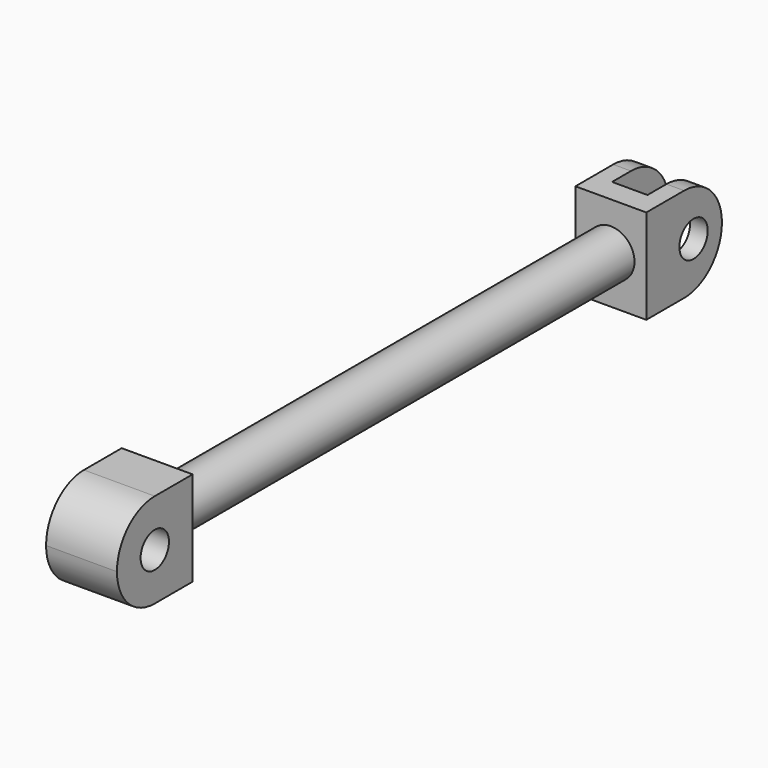
from build123d import *

# Parameters (mm, degrees)
F0_R      = 12.7
F1_DEPTH  = 304.8
F2_W      = 38.1
F2_H      = 50.8
F3_DEPTH  = 50.8
F4_R      = 9.525
F5_DEPTH  = 38.101
F6_W      = 38.1
F6_H      = 50.8
F7_DEPTH  = 50.8
F8_W      = 19.05
F8_H      = 50.8
F9_DEPTH  = 38.1
F10_R     = 9.525
F11_DEPTH = 38.101
F12_R     = 25.39999


# Not quite as in the source:
# - a fillet or chamfer is up to 0.001 mm smaller than in the source, because OpenCascade refuses the exact size


with BuildPart() as f1:
    # F0 (on Front) → F1 (new body)
    with BuildSketch(Plane.XZ):
        Circle(F0_R)
    extrude(amount=F1_DEPTH)

    # F2 (on face) → F3 (join)
    with BuildSketch(Plane.XZ.offset(304.8)):
        Rectangle(F2_W, F2_H)
    extrude(amount=F3_DEPTH)

    # F4 (on face) → F5 (cut, through all)
    with BuildSketch(Plane(origin=(-19.05, 0, 0), x_dir=(0, -1, 0), z_dir=(-1, 0, 0))):
        with Locations((330.2, 0)):
            Circle(F4_R)
    extrude(amount=-F5_DEPTH, mode=Mode.SUBTRACT)

    # F6 (on face) → F7 (join)
    with BuildSketch(Plane(origin=(0, 0, 0), x_dir=(-1, 0, 0), z_dir=(0, 1, 0))):
        Rectangle(F6_W, F6_H)
    extrude(amount=F7_DEPTH)

    # F8 (on face) → F9 (cut)
    with BuildSketch(Plane(origin=(0, 50.8, 0), x_dir=(-1, 0, 0), z_dir=(0, 1, 0))):
        Rectangle(F8_W, F8_H)
    extrude(amount=-F9_DEPTH, mode=Mode.SUBTRACT)

    # F10 (on face) → F11 (cut, through all)
    with BuildSketch(Plane.YZ.offset(19.05)):
        with Locations((31.75, 0)):
            Circle(F10_R)
    extrude(amount=-F11_DEPTH, mode=Mode.SUBTRACT)

    # F12 (radius 25.4 in the source; OpenCascade refuses exactly that, so slightly less here)
    f12_edges = [f1.edges().sort_by_distance(p)[0] for p in [
        (14.2875, 50.8, 25.4),
        (14.2875, 50.8, -25.4),
        (-14.2875, 50.8, -25.4),
        (-14.2875, 50.8, 25.4),
        (0, -355.6, 25.4),
        (0, -355.6, -25.4),
    ]]
    fillet(f12_edges, radius=F12_R)


solid = f1.part
